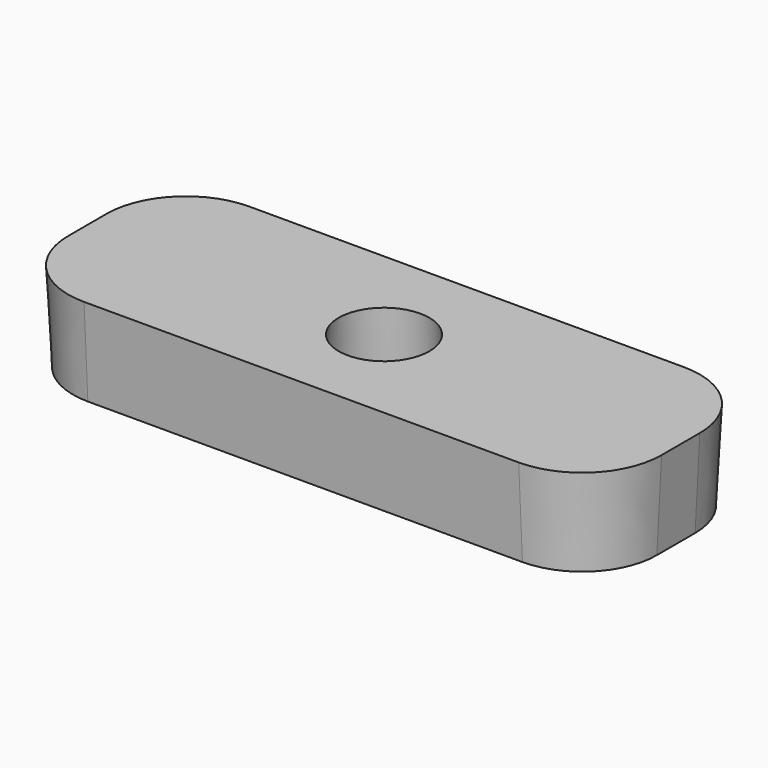
from build123d import *

# Parameters (mm, degrees)
F0_R                   = 3.35
F1_DEPTH               = 6
DRAFT_F1_DRAFTED_ANGLE = -3
F2_R                   = 3.0355533243
F3_DEPTH               = 4.15
F3_TAPER               = 3


# Not quite as in the source:
# - an extrude with a draft is written as a straight extrude whose walls are then drafted


with BuildPart() as f1:
    # F0 (on Top) → F1 (new body)
    with BuildSketch(Plane.XY):
        with BuildLine():
            Line((-12.75, 6.6), (-14.55, 6.6))
            ThreePointArc((-14.55, 6.6), (-18.0855339059, 5.1355339059), (-19.55, 1.6))
            Line((-19.55, 1.6), (-19.55, -1.6))
            ThreePointArc((-19.55, -1.6), (-18.0855339059, -5.1355339059), (-14.55, -6.6))
            Line((-14.55, -6.6), (-12.75, -6.6))
            Line((-12.75, -6.6), (12.75, -6.6))
            Line((12.75, -6.6), (14.55, -6.6))
            ThreePointArc((14.55, -6.6), (18.0855339059, -5.1355339059), (19.55, -1.6))
            Line((19.55, -1.6), (19.55, 1.6))
            ThreePointArc((19.55, 1.6), (18.0855339059, 5.1355339059), (14.55, 6.6))
            Line((14.55, 6.6), (12.75, 6.6))
            Line((12.75, 6.6), (-12.75, 6.6))
        make_face()
        with BuildLine():
            ThreePointArc((-17.75, 0.45), (-16.2855339059, 3.9855339059), (-12.75, 5.45))
            Line((-12.75, 5.45), (-5.2610003802, 5.45))
            Line((-5.2610003802, 5.45), (5.2610003802, 5.45))
            Line((5.2610003802, 5.45), (12.75, 5.45))
            ThreePointArc((12.75, 5.45), (16.2855339059, 3.9855339059), (17.75, 0.45))
            Line((17.75, 0.45), (17.75, -0.45))
            ThreePointArc((17.75, -0.45), (16.2855339059, -3.9855339059), (12.75, -5.45))
            Line((12.75, -5.45), (5.2610003802, -5.45))
            Line((5.2610003802, -5.45), (-5.2610003802, -5.45))
            Line((-5.2610003802, -5.45), (-12.75, -5.45))
            ThreePointArc((-12.75, -5.45), (-16.2855339059, -3.9855339059), (-17.75, -0.45))
            Line((-17.75, -0.45), (-17.75, 0.45))
        make_face(mode=Mode.SUBTRACT)
        with BuildLine():
            Line((5.2610003802, 5.45), (-5.2610003802, 5.45))
            ThreePointArc((-5.2610003802, 5.45), (-7.575, 0), (-5.2610003802, -5.45))
            Line((-5.2610003802, -5.45), (5.2610003802, -5.45))
            ThreePointArc((5.2610003802, -5.45), (7.575, 0), (5.2610003802, 5.45))
        make_face()
        Circle(F0_R, mode=Mode.SUBTRACT)
    extrude(amount=F1_DEPTH)

    # draft_F1_drafted
    draft_f1_drafted_walls = [f1.faces().sort_by_distance(p)[0] for p in [
        (18.0855339059, 5.1355339059, 4),
        (0, 6.6, 4),
        (-18.0855339059, 5.1355339059, 4),
        (-19.55, 0, 4),
        (-18.0855339059, -5.1355339059, 4),
        (0, -6.6, 4),
        (18.0855339059, -5.1355339059, 4),
        (19.55, 0, 4),
        (16.2855339059, -3.9855339059, 4),
        (9.0055001901, -5.45, 4),
        (7.575, 0, 4),
        (9.0055001901, 5.45, 4),
        (16.2855339059, 3.9855339059, 4),
        (17.75, 0, 4),
        (-9.0055001901, -5.45, 4),
        (-16.2855339059, -3.9855339059, 4),
        (-17.75, 0, 4),
        (-16.2855339059, 3.9855339059, 4),
        (-9.0055001901, 5.45, 4),
        (-7.575, 0, 4),
        (-3.35, 0, 4),
    ]]
    draft(draft_f1_drafted_walls, neutral_plane=Plane.XY, angle=DRAFT_F1_DRAFTED_ANGLE)

    # F2 (on face) → F3 (join)
    with BuildSketch(Plane.XY.offset(6)):
        with BuildLine():
            ThreePointArc((-19.8644466757, -1.6), (-18.3078812826, -5.3578812826), (-14.55, -6.9144466757))
            Line((-14.55, -6.9144466757), (14.55, -6.9144466757))
            ThreePointArc((14.55, -6.9144466757), (18.3078812826, -5.3578812826), (19.8644466757, -1.6))
            Line((19.8644466757, -1.6), (19.8644466757, 1.6))
            ThreePointArc((19.8644466757, 1.6), (18.3078812826, 5.3578812826), (14.55, 6.9144466757))
            Line((14.55, 6.9144466757), (-14.55, 6.9144466757))
            ThreePointArc((-14.55, 6.9144466757), (-18.3078812826, 5.3578812826), (-19.8644466757, 1.6))
            Line((-19.8644466757, 1.6), (-19.8644466757, -1.6))
        make_face()
        with BuildLine():
            ThreePointArc((-17.4355533243, 0.45), (-16.0631865292, 3.7631865292), (-12.75, 5.1355533243))
            Line((-12.75, 5.1355533243), (-5.9891118625, 5.1355533243))
            ThreePointArc((-5.9891118625, 5.1355533243), (-7.8894466757, 0), (-5.9891118625, -5.1355533243))
            Line((-5.9891118625, -5.1355533243), (-12.75, -5.1355533243))
            ThreePointArc((-12.75, -5.1355533243), (-16.0631865292, -3.7631865292), (-17.4355533243, -0.45))
            Line((-17.4355533243, -0.45), (-17.4355533243, 0.45))
        make_face(mode=Mode.SUBTRACT)
        Circle(F2_R, mode=Mode.SUBTRACT)
        with BuildLine():
            Line((12.75, -5.1355533243), (5.9891118625, -5.1355533243))
            ThreePointArc((5.9891118625, -5.1355533243), (7.8894466757, 0), (5.9891118625, 5.1355533243))
            Line((5.9891118625, 5.1355533243), (12.75, 5.1355533243))
            ThreePointArc((12.75, 5.1355533243), (16.0631865292, 3.7631865292), (17.4355533243, 0.45))
            Line((17.4355533243, 0.45), (17.4355533243, -0.45))
            ThreePointArc((17.4355533243, -0.45), (16.0631865292, -3.7631865292), (12.75, -5.1355533243))
        make_face(mode=Mode.SUBTRACT)
        with BuildLine():
            Line((-5.9891118625, 5.1355533243), (-12.75, 5.1355533243))
            ThreePointArc((-12.75, 5.1355533243), (-16.0631865292, 3.7631865292), (-17.4355533243, 0.45))
            Line((-17.4355533243, 0.45), (-17.4355533243, -0.45))
            ThreePointArc((-17.4355533243, -0.45), (-16.0631865292, -3.7631865292), (-12.75, -5.1355533243))
            Line((-12.75, -5.1355533243), (-5.9891118625, -5.1355533243))
            ThreePointArc((-5.9891118625, -5.1355533243), (-7.8894466757, 0), (-5.9891118625, 5.1355533243))
        make_face()
        with BuildLine():
            ThreePointArc((5.9891118625, 5.1355533243), (7.8894466757, 0), (5.9891118625, -5.1355533243))
            Line((5.9891118625, -5.1355533243), (12.75, -5.1355533243))
            ThreePointArc((12.75, -5.1355533243), (16.0631865292, -3.7631865292), (17.4355533243, -0.45))
            Line((17.4355533243, -0.45), (17.4355533243, 0.45))
            ThreePointArc((17.4355533243, 0.45), (16.0631865292, 3.7631865292), (12.75, 5.1355533243))
            Line((12.75, 5.1355533243), (5.9891118625, 5.1355533243))
        make_face()
    extrude(amount=-F3_DEPTH, taper=F3_TAPER)


solid = f1.part
